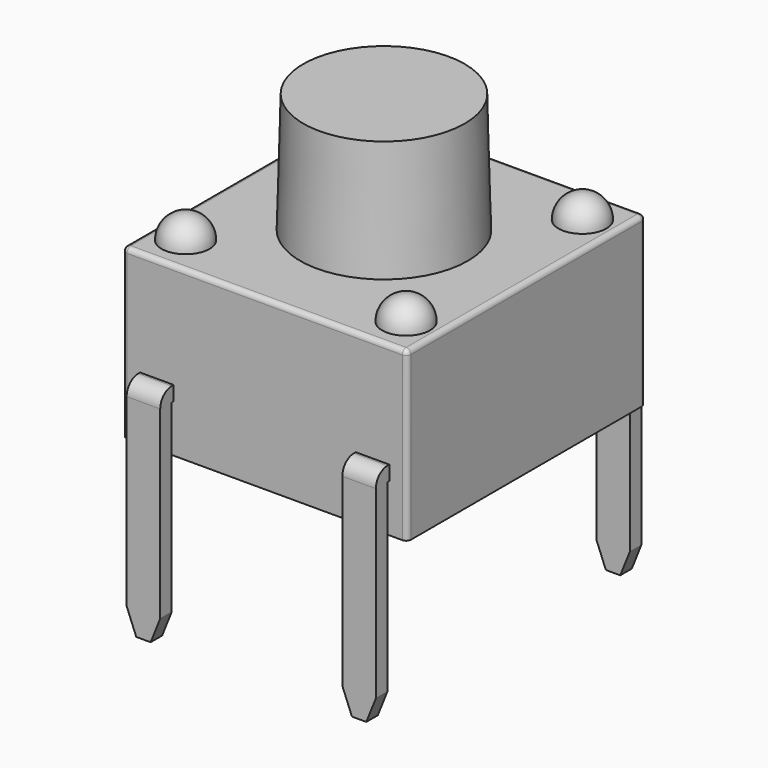
from build123d import *

# Parameters (mm, degrees)
F0_W        = 5.9436
F0_H        = 6.223
F1_DEPTH    = 3.5
F2_R        = 1.75
F3_DEPTH    = 2.5
F3_TAPER    = 1.5
F4_R        = 0.1
F5_R        = 0.5
F6_DEPTH    = 0.5
F7_R        = 0.49999
F8_W        = 0.7
F8_H        = 0.3
F11_SIZE2   = 0.5
F11_SIZE    = 0.2
F11_2_SIZE2 = 0.5
F11_2_SIZE  = 0.2


# Not quite as in the source:
# - a fillet or chamfer is up to 0.001 mm smaller than in the source, because OpenCascade refuses the exact size


with BuildPart() as f1:
    # F0 (on Top) → F1 (new body)
    with BuildSketch(Plane.XY):
        Rectangle(F0_W, F0_H)
    extrude(amount=F1_DEPTH)

    # F2 (on face) → F3 (join)
    with BuildSketch(Plane.XY.offset(3.5)):
        Circle(F2_R)
    extrude(amount=F3_DEPTH, taper=F3_TAPER)

    # F4
    f4_edges = [f1.edges().sort_by_distance(p)[0] for p in [
        (2.9718, -3.1115, 1.75),
        (-2.9718, -3.1115, 1.75),
        (-2.9718, 3.1115, 1.75),
        (2.9718, 3.1115, 1.75),
        (2.9718, 0, 3.5),
        (0, -3.1115, 3.5),
        (-2.9718, 0, 3.5),
        (0, 3.1115, 3.5),
    ]]
    fillet(f4_edges, radius=F4_R)

    # F5 (on face) → F6 (join)
    with BuildSketch(Plane.XY.offset(3.5)):
        with Locations((2.3, -2.3)):
            Circle(F5_R)
        with Locations((2.3, 2.3)):
            Circle(F5_R)
        with Locations((-2.3, 2.3)):
            Circle(F5_R)
        with Locations((-2.3, -2.3)):
            Circle(F5_R)
    extrude(amount=F6_DEPTH)

    # F7 (radius 0.5 in the source; OpenCascade refuses exactly that, so slightly less here)
    f7_edges = [f1.edges().sort_by_distance(p)[0] for p in [
        (1.8, -2.3, 4),
        (1.8, 2.3, 4),
        (-2.8, 2.3, 4),
        (-2.8, -2.3, 4),
    ]]
    fillet(f7_edges, radius=F7_R)

    # F10: sweep along a path in F9
    with BuildLine(Plane.YZ) as f10_path:
        Line((-3.1115, 1.15), (-3.1615, 1.15))
        ThreePointArc((-3.1615, 1.15), (-3.2675660172, 1.1060660172), (-3.3115, 1))
        Line((-3.3115, 1), (-3.3115, -3.35))
    # F8 (on face) → F10 (sweep)
    with BuildSketch(Plane.XZ.offset(3.1115)):
        with Locations((-2.25, 1.15)):
            Rectangle(F8_W, F8_H)
        with Locations((2.25, 1.15)):
            Rectangle(F8_W, F8_H)
    sweep(path=f10_path.line)

    # F11
    f11_edges = [f1.edges().sort_by_distance(p)[0] for p in [
        (-2.6, -3.3115, -3.35),
        (-1.9, -3.3115, -3.35),
    ]]
    f11_side = f1.faces().sort_by_distance((-2.25, -3.3115, -3.35))[0]
    chamfer(f11_edges, length=F11_SIZE, length2=F11_SIZE2, reference=f11_side)

    # F11#2
    f11_2_edges = [f1.edges().sort_by_distance(p)[0] for p in [
        (1.9, -3.3115, -3.35),
        (2.6, -3.3115, -3.35),
    ]]
    f11_2_side = f1.faces().sort_by_distance((2.25, -3.3115, -3.35))[0]
    chamfer(f11_2_edges, length=F11_2_SIZE, length2=F11_2_SIZE2, reference=f11_2_side)

    # F12: F1 across plane


with BuildPart() as f1_1:
    add(f1.part)
    add(f1.part.mirror(Plane.XZ))


solid = f1_1.part
